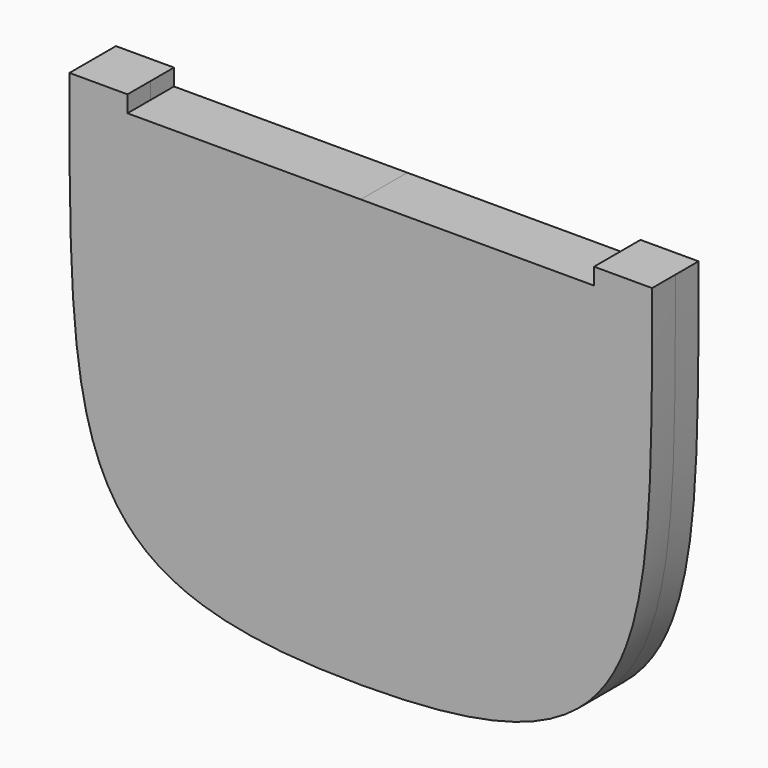
from build123d import *

# Parameters (mm, degrees)
F1_DEPTH = 5


# Not quite as in the source:
# - ends of sketch curves that miss each other by under 0.0002 mm in the source are joined
# - the dataset's text gives a spline's control points without its knots; the knots are read off the source's solid


with BuildPart() as f1:
    # F0 (on Front) → F1 (new body, symmetric)
    with BuildSketch(Plane.XZ):
        with BuildLine():
            add(Edge.make_bspline(
                [(0, 0), (-50.185825198, 0), (-50.185825198, 18.9878194471), (-50.185825198, 76.5)],
                knots=[0, 0, 0, 0, 91.4924425884, 91.4924425884, 91.4924425884, 91.4924425884], degree=3))
            Line((0, 0), (0, 10))
            add(Edge.make_bspline(
                [(0, 10), (-2.9789681379, 10), (-8.4955397739, 10.1413450921), (-15.4737654621, 10.776664129), (-21.1789329484, 11.809227477), (-25.6521730863, 13.1752084964), (-29.0027084757, 14.7778973307), (-31.4729254896, 16.5529365311), (-33.4126965241, 18.598166324), (-35.0926907472, 21.1958365208), (-36.5807802286, 24.6299720269), (-37.8303704724, 29.0468893658), (-38.7969863936, 34.4792506235), (-39.4760376196, 40.9128537432), (-39.8974470799, 48.3258672411), (-40.1654290193, 58.7432213291), (-40.1839080708, 67.5582061549), (-40.185555974, 73.6273912162)],
                knots=[0, 0, 0, 0, 0.0625, 0.125, 0.1875, 0.25, 0.3125, 0.375, 0.4375, 0.5, 0.5625, 0.625, 0.6875, 0.75, 0.8125, 0.875, 0.9831466803, 0.9831466803, 0.9831466803, 0.9831466803], degree=3))
            add(Edge.make_bspline(
                [(-40.185555974, 73.6273912162), (-40.1858125489, 74.5723499258), (-40.1858251755, 75.529010691), (-40.1858251979, 76.4973911991)],
                knots=[0.9831466803, 0.9831466803, 0.9831466803, 0.9831466803, 0.9999848796, 0.9999848796, 0.9999848796, 0.9999848796], degree=3))
            Line((-40.185825198, 76.4973911982), (-50.185825198, 76.5))
        make_face()
        with BuildLine():
            Line((0, 10), (0, 0))
            add(Edge.make_bspline(
                [(0, 0), (50.185825198, 0), (50.185825198, 18.9878194471), (50.185825198, 76.5)],
                knots=[0, 0, 0, 0, 91.4924425884, 91.4924425884, 91.4924425884, 91.4924425884], degree=3))
            Line((50.185825198, 76.5), (40.185825198, 76.5))
            add(Edge.make_bspline(
                [(40.185555974, 73.6273912083), (40.1858127793, 74.5731984789), (40.185825198, 75.5307288311), (40.185825198, 76.5)],
                knots=[0.9831466802, 0.9831466802, 0.9831466802, 0.9831466802, 1, 1, 1, 1], degree=3))
            add(Edge.make_bspline(
                [(0, 10), (2.9789681379, 10), (8.4955397739, 10.1413450921), (15.4737654621, 10.776664129), (21.1789329484, 11.809227477), (25.6521730863, 13.1752084964), (29.0027084757, 14.7778973307), (31.4729254896, 16.5529365311), (33.4126965241, 18.598166324), (35.0926907472, 21.1958365208), (36.5807802286, 24.6299720269), (37.8303704724, 29.0468893658), (38.7969863936, 34.4792506235), (39.4760376196, 40.9128537432), (39.8974470799, 48.3258672411), (40.1654290192, 58.7432213269), (40.1839080707, 67.55820615), (40.185555974, 73.6273912083)],
                knots=[0, 0, 0, 0, 0.0625, 0.125, 0.1875, 0.25, 0.3125, 0.375, 0.4375, 0.5, 0.5625, 0.625, 0.6875, 0.75, 0.8125, 0.875, 0.9831466802, 0.9831466802, 0.9831466802, 0.9831466802], degree=3))
        make_face()
        with BuildLine():
            add(Edge.make_bspline(
                [(0, 10), (-2.9789681379, 10), (-8.4955397739, 10.1413450921), (-15.4737654621, 10.776664129), (-21.1789329484, 11.809227477), (-25.6521730863, 13.1752084964), (-29.0027084757, 14.7778973307), (-31.4729254896, 16.5529365311), (-33.4126965241, 18.598166324), (-35.0926907472, 21.1958365208), (-36.5807802286, 24.6299720269), (-37.8303704724, 29.0468893658), (-38.7969863936, 34.4792506235), (-39.4760376196, 40.9128537432), (-39.8974470799, 48.3258672411), (-40.1654290193, 58.7432213291), (-40.1839080708, 67.5582061549), (-40.185555974, 73.6273912162)],
                knots=[0, 0, 0, 0, 0.0625, 0.125, 0.1875, 0.25, 0.3125, 0.375, 0.4375, 0.5, 0.5625, 0.625, 0.6875, 0.75, 0.8125, 0.875, 0.9831466803, 0.9831466803, 0.9831466803, 0.9831466803], degree=3))
            Line((0, 10), (0, 73.6273912083))
            Line((0, 73.6273912083), (-40.185555974, 73.6273912162))
        make_face()
        with BuildLine():
            Line((0, 73.6273912083), (0, 10))
            add(Edge.make_bspline(
                [(0, 10), (2.9789681379, 10), (8.4955397739, 10.1413450921), (15.4737654621, 10.776664129), (21.1789329484, 11.809227477), (25.6521730863, 13.1752084964), (29.0027084757, 14.7778973307), (31.4729254896, 16.5529365311), (33.4126965241, 18.598166324), (35.0926907472, 21.1958365208), (36.5807802286, 24.6299720269), (37.8303704724, 29.0468893658), (38.7969863936, 34.4792506235), (39.4760376196, 40.9128537432), (39.8974470799, 48.3258672411), (40.1654290192, 58.7432213269), (40.1839080707, 67.55820615), (40.185555974, 73.6273912083)],
                knots=[0, 0, 0, 0, 0.0625, 0.125, 0.1875, 0.25, 0.3125, 0.375, 0.4375, 0.5, 0.5625, 0.625, 0.6875, 0.75, 0.8125, 0.875, 0.9831466802, 0.9831466802, 0.9831466802, 0.9831466802], degree=3))
            Line((40.185555974, 73.6273912083), (0, 73.6273912083))
        make_face()
    extrude(amount=F1_DEPTH, both=True)


solid = f1.part
